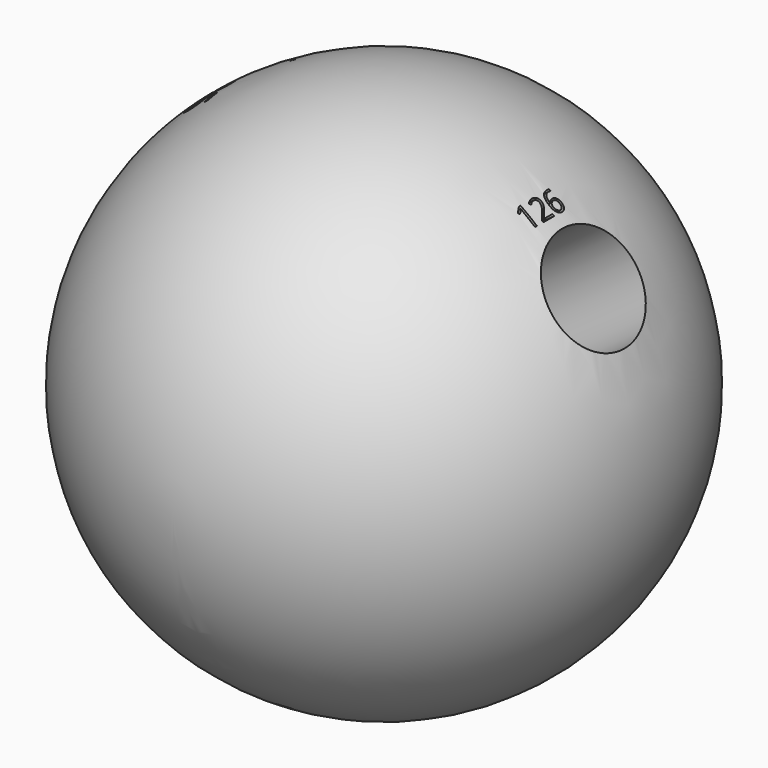
from build123d import *

# Parameters (mm, degrees)
F4_R          = 3.175
F5_DEPTH      = 25.4
F7_TEXT_SIZE  = 1.7962787145
F8_DEPTH      = 10.16
F10_ANGLE     = 125
F12_TEXT_SIZE = 2.6581647237
F13_DEPTH     = 10.16
F15_ANGLE     = 126
F17_TEXT_SIZE = 1.6740775512
F18_DEPTH     = 10.16


# Not quite as in the source:
# - Text() gives the source's letters only with a copy of the font that has no kerning and outlines rounded to 1/6400 em; it was checked with that copy


with BuildPart() as f2:
    # F0 (on Right) → F2 (revolve)
    with BuildSketch(Plane.YZ):
        with BuildLine():
            Line((15.875, 0), (-15.875, 0))
            ThreePointArc((-15.875, 0), (0, -15.875), (15.875, 0))
        make_face()
    revolve(axis=Axis((0, 0, 0), (0, -1, 0)))

    # F7 (on offset) → F8 (cut)
    with BuildSketch(Plane(origin=(0, 0, -19.05), x_dir=(1, 0, 0), z_dir=(0, 0, -1))):
        with Locations((-1.480293402, 3.3147567883)):
            Text('109', F7_TEXT_SIZE, font='Open Sans', text_align=(TextAlign.LEFT, TextAlign.BOTTOM))
    extrude(amount=-F8_DEPTH, mode=Mode.SUBTRACT)

    # F12 (on offset) → F13 (cut)
    with BuildSketch(Plane(origin=(-15.6048464437, 0, 10.9266311125), x_dir=(0, -1, 0), z_dir=(-0.8191520443, 0, 0.5735764364))):
        with Locations((-2.1189313848, 3.5988120362)):
            Text('125', F12_TEXT_SIZE, font='Open Sans', text_align=(TextAlign.LEFT, TextAlign.BOTTOM))
    extrude(amount=-F13_DEPTH, mode=Mode.SUBTRACT)

    # F17 (on offset) → F18 (cut)
    with BuildSketch(Plane(origin=(15.4117737428, 0, 11.1973090562), x_dir=(0, 1, 0), z_dir=(0.8090169944, 0, 0.5877852523))):
        with Locations((-1.7781956849, 3.8627684116)):
            Text('126', F17_TEXT_SIZE, font='Open Sans', text_align=(TextAlign.LEFT, TextAlign.BOTTOM))
    extrude(amount=-F18_DEPTH, mode=Mode.SUBTRACT)


with BuildPart() as f5:
    # F4 (on offset) → F5 (new body)
    with BuildSketch(Plane.XY.offset(-6.35)):
        Circle(F4_R)
    extrude(amount=-F5_DEPTH)


with BuildPart() as f10_1:
    # F10: copy of F5
    add(f5.part.rotate(Axis((0, -8.5725020617, 0), (0, 1, 0)), F10_ANGLE))


with BuildPart() as f15_1:
    # F15: copy of F5
    add(f5.part.rotate(Axis((0, -2.3966133595, 0), (0, -1, 0)), F15_ANGLE))


with BuildPart() as f2_1:
    add(f2.part)

    # F19: cut F10_1, F5, F15_1
    add(f10_1.part, mode=Mode.SUBTRACT)
    add(f5.part, mode=Mode.SUBTRACT)
    add(f15_1.part, mode=Mode.SUBTRACT)


solid = f2_1.part
